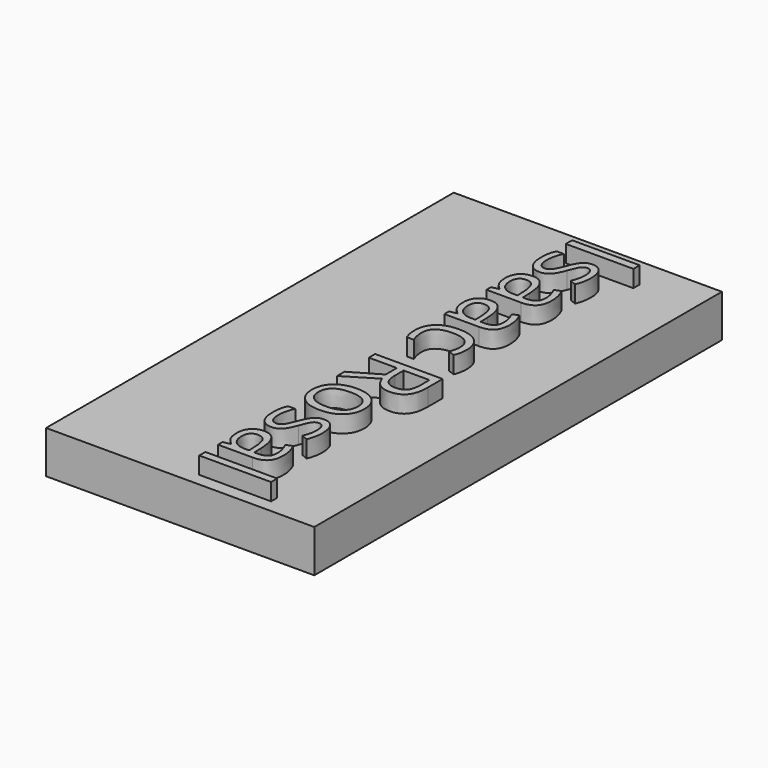
from build123d import *

# Parameters (mm, degrees)
F0_W         = 20.0071665458
F0_H         = 38.010796532
F1_DEPTH     = 3.175
F2_TEXT_SIZE = 7.0555555556
F3_DEPTH     = 1.27


# Not quite as in the source:
# - Text() gives the source's letters only with a copy of the font that has no kerning and outlines rounded to 1/6400 em; it was checked with that copy


with BuildPart() as f1:
    # F0 (on Top) → F1 (new body)
    with BuildSketch(Plane.XY):
        with Locations((-5.7405310217, -0.5519213155)):
            Rectangle(F0_W, F0_H)
    extrude(amount=F1_DEPTH)

    # F2 (on face) → F3 (join)
    with BuildSketch(Plane.XY.offset(3.175)):
        with Locations(Location((-5.08, 16.8571908799), (0, 0, -90))):
            Text('Isaac Rosal', F2_TEXT_SIZE, font='Open Sans', text_align=(TextAlign.LEFT, TextAlign.BOTTOM))
    extrude(amount=F3_DEPTH)


solid = f1.part
